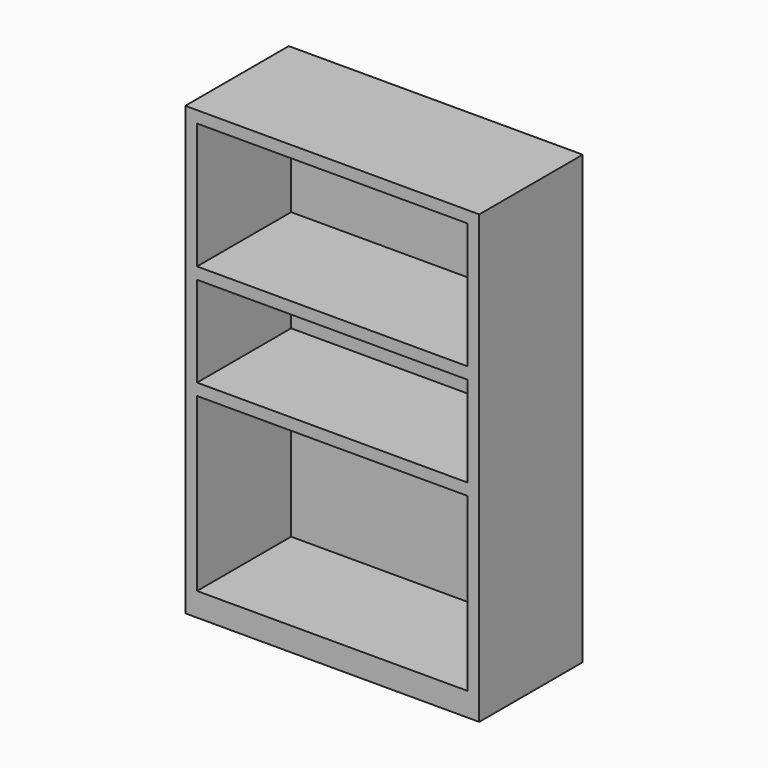
from build123d import *

# Parameters (mm, degrees)
F0_W     = 25
F0_H     = 38
F0_W_2   = 22.9999984503
F0_H_2   = 15.5999984503
F0_H_3   = 7.7
F0_H_4   = 10.7
F1_DEPTH = 10
F2_W     = 25
F2_H     = 38
F2_W_2   = 22.9999984503
F2_H_2   = 15.5999984503
F2_H_3   = 7.7
F2_H_4   = 10.7
F3_DEPTH = 1
F4_DEPTH = 1
F5_W     = 23.0000000447
F5_H     = 9.0000000447
F6_DEPTH = 1


with BuildPart() as f1:
    # F0 (on Front) → F1 (new body)
    with BuildSketch(Plane.XZ):
        Rectangle(F0_W, F0_H)
        with Locations((0, -10.2)):
            Rectangle(F0_W_2, F0_H_2, mode=Mode.SUBTRACT)
        with Locations((0, 2.4499992251)):
            Rectangle(F0_W_2, F0_H_3, mode=Mode.SUBTRACT)
        with Locations((0, 12.6499992251)):
            Rectangle(F0_W_2, F0_H_4, mode=Mode.SUBTRACT)
    extrude(amount=F1_DEPTH)

    # F2 (on face) → F3 (join)
    with BuildSketch(Plane(origin=(0, 0, 0), x_dir=(-1, 0, 0), z_dir=(0, 1, 0))):
        Rectangle(F2_W, F2_H)
        with Locations((0, -10.2)):
            Rectangle(F2_W_2, F2_H_2, mode=Mode.SUBTRACT)
        with Locations((0, 2.4499992251)):
            Rectangle(F2_W_2, F2_H_3, mode=Mode.SUBTRACT)
        with Locations((0, 12.6499992251)):
            Rectangle(F2_W_2, F2_H_4, mode=Mode.SUBTRACT)
        with Locations((0, -10.2)):
            Rectangle(F2_W_2, F2_H_2)
        with Locations((0, 12.6499992251)):
            Rectangle(F2_W_2, F2_H_4)
        with Locations((0, 2.4499992251)):
            Rectangle(F2_W_2, F2_H_3)
    extrude(amount=F3_DEPTH)

    # F4 (add): a face of the model
    f4_faces = [f1.faces().sort_by_distance(p)[0] for p in [
        (0, -5, -17.9999992251),
    ]]
    extrude(f4_faces, amount=F4_DEPTH)

    # F5 (on face) → F6 (cut)
    with BuildSketch(Plane(origin=(0, 0, -19), x_dir=(1, 0, 0), z_dir=(0, 0, -1))):
        with Locations((0, 4.5)):
            Rectangle(F5_W, F5_H)
    extrude(amount=-F6_DEPTH, mode=Mode.SUBTRACT)


solid = f1.part
